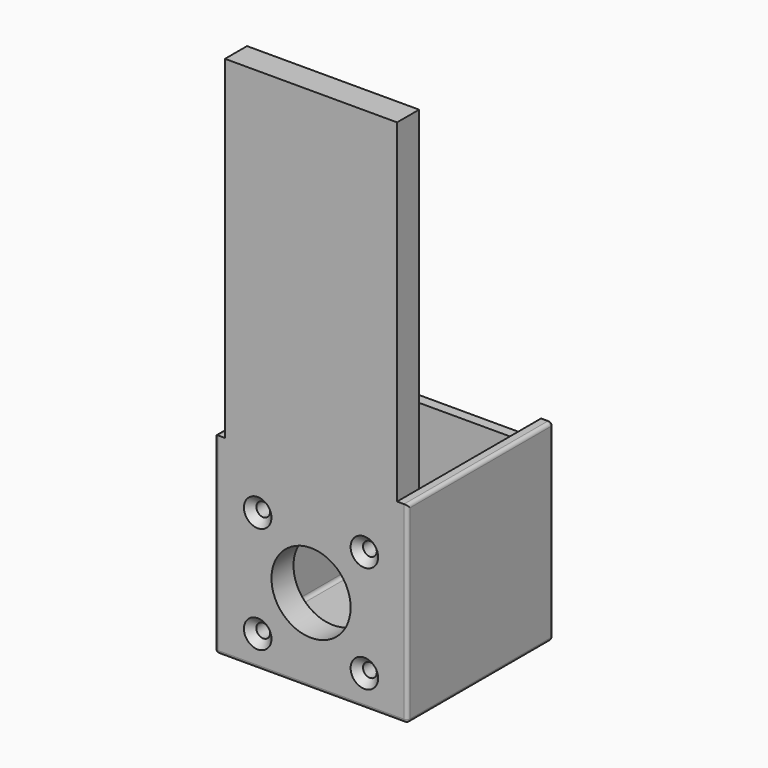
from build123d import *

# Parameters (mm, degrees)
F0_W      = 50
F0_H      = 150
F0_R      = 2
F0_R_2    = 11.5
F1_DEPTH  = 8
F2_SIZE   = 2
F3_W      = 50
F3_H      = 53
F4_DEPTH  = 3
F5_W      = 50
F5_H      = 53
F6_DEPTH  = 3
F7_W      = 56
F7_H      = 50
F8_DEPTH  = 3
F9_W      = 56
F9_H      = 56
F10_DEPTH = 3
F11_R     = 1
F13_DEPTH = 45


with BuildPart() as f1:
    # F0 (on Front) → F1 (new body)
    with BuildSketch(Plane.XZ):
        with Locations((25, 75)):
            Rectangle(F0_W, F0_H)
        with Locations((9.5, 6)):
            Circle(F0_R, mode=Mode.SUBTRACT)
        with Locations((9.5, 37)):
            Circle(F0_R, mode=Mode.SUBTRACT)
        with Locations((25, 21.5)):
            Circle(F0_R_2, mode=Mode.SUBTRACT)
        with Locations((40.5, 6)):
            Circle(F0_R, mode=Mode.SUBTRACT)
        with Locations((40.5, 37)):
            Circle(F0_R, mode=Mode.SUBTRACT)
    extrude(amount=F1_DEPTH)

    # F2
    f2_edges = [f1.edges().sort_by_distance(p)[0] for p in [
        (7.5, -8, 37),
        (38.5, -8, 37),
        (38.5, -8, 6),
        (7.5, -8, 6),
    ]]
    chamfer(f2_edges, length=F2_SIZE)

    # F3 (on face) → F4 (join)
    with BuildSketch(Plane.YZ.offset(50)):
        with Locations((17, 26.5)):
            Rectangle(F3_W, F3_H)
    extrude(amount=F4_DEPTH)

    # F5 (on face) → F6 (join)
    with BuildSketch(Plane(origin=(0, 0, 0), x_dir=(0, -1, 0), z_dir=(-1, 0, 0))):
        with Locations((-17, 26.5)):
            Rectangle(F5_W, F5_H)
    extrude(amount=F6_DEPTH)

    # F7 (on face) → F8 (join)
    with BuildSketch(Plane(origin=(0, 0, 0), x_dir=(1, 0, 0), z_dir=(0, 0, -1))):
        with Locations((25, -17)):
            Rectangle(F7_W, F7_H)
    extrude(amount=F8_DEPTH)

    # F9 (on face) → F10 (join)
    with BuildSketch(Plane(origin=(0, 42, 0), x_dir=(-1, 0, 0), z_dir=(0, 1, 0))):
        with Locations((-25, 25)):
            Rectangle(F9_W, F9_H)
    extrude(amount=F10_DEPTH)

    # F11
    f11_edges = [f1.edges().sort_by_distance(p)[0] for p in [
        (50, 0, 26.5),
        (25, 0, 0),
        (50, 21, 0),
        (0, 21, 0),
        (0, 42, 26.5),
        (50, 42, 26.5),
        (0, 0, 26.5),
        (25, 42, 0),
        (53, 45, 25),
        (25, 45, 53),
        (25, 45, -3),
        (-3, 45, 25),
        (25, -8, -3),
        (-3, 18.5, -3),
        (53, 18.5, -3),
        (53, -8, 25),
        (53, 18.5, 53),
        (-3, -8, 25),
        (-3, 18.5, 53),
    ]]
    fillet(f11_edges, radius=F11_R)

    # F12 (on face) → F13 (cut, through all)
    with BuildSketch(Plane(origin=(0, 45, 0), x_dir=(-1, 0, 0), z_dir=(0, 1, 0))):
        Polygon((-50, 50.1), (-51, 50.1), (-51, 47), (1, 47), (1, 50.1), (-1, 50.1), (-1, 53), (-50, 53), align=None)
    extrude(amount=-F13_DEPTH, mode=Mode.SUBTRACT)


solid = f1.part
